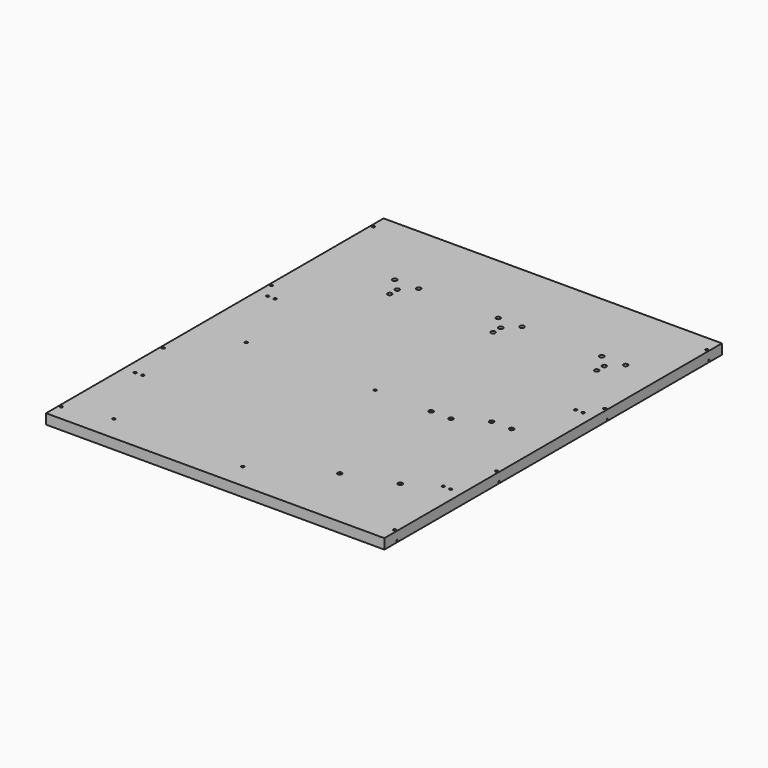
from build123d import *

# Parameters (mm, degrees)
F0_W            = 425
F0_H            = 530
F1_DEPTH        = 6.35
F3_D            = 3.3
F3_CBORE_D      = 6.5
F3_CBORE_DEPTH  = 3
F5_D            = 5.5
F5_CBORE_D      = 9.75
F5_CBORE_DEPTH  = 5
F7_D            = 3.3
F7_CBORE_D      = 6.5
F7_CBORE_DEPTH  = 3
F9_D            = 5.5
F9_DEPTH        = 1
F9_TIP          = 1.6523667023
F11_D           = 3.3
F11_CBORE_D     = 6.5
F11_CBORE_DEPTH = 3


# Not quite as in the source:
# - a feature names something its author has since deleted; it is built from what else it names


with BuildPart() as f1:
    # F0 (on Top) → F1 (new body, symmetric)
    with BuildSketch(Plane.XY):
        Rectangle(F0_W, F0_H)
    extrude(amount=F1_DEPTH, both=True)

    # F3 (through all)
    with Locations(Plane(origin=(0, 0, -6.35), x_dir=(1, 0, 0), z_dir=(0, 0, -1))):
        with Locations((-209.325, 245), (-209.325, 85), (-209.325, -85), (-209.325, -245), (209.325, -245), (209.325, -85), (209.325, 85), (209.325, 245), (-198.2, 143), (-188.7, 143), (198.2, 143), (188.7, 143), (-198.2, -65), (-188.7, -65), (188.7, -65), (198.2, -65)):
            CounterBoreHole(F3_D / 2, F3_CBORE_D / 2, F3_CBORE_DEPTH)

    # F5 (through all)
    with Locations(Plane(origin=(0, 0, -6.35), x_dir=(1, 0, 0), z_dir=(0, 0, -1))):
        with Locations((-122.5, -170), (-92.5, -170), (-107.5, -155.235), (-107.5, -143.235), (167.5, -170), (152.5, -155.235), (152.5, -143.235), (137.5, -170), (37.5, -170), (7.5, -170), (22.5, -155.235), (22.5, -143.235)):
            CounterBoreHole(F5_D / 2, F5_CBORE_D / 2, F5_CBORE_DEPTH)

    # F7 (through all)
    with Locations(Plane(origin=(0, 0, -6.35), x_dir=(1, 0, 0), z_dir=(0, 0, -1))):
        with Locations((152.5, 165), (165, 6), (140, 6), (92.5, 185), (105, 26), (80, 26)):
            CounterBoreHole(F7_D / 2, F7_CBORE_D / 2, F7_CBORE_DEPTH)

    # F9
    with Locations(Plane.XY.offset(6.35)):
        with Locations((165, -6), (140, -6), (105, -26), (105, -26), (80, -26), (152.5, -165), (92.5, -185)):
            Hole(F9_D / 2, depth=F9_DEPTH)
            with Locations((0, 0, -(F9_DEPTH + F9_TIP / 2))):  # 118° drill point
                Cone(0, F9_D / 2, F9_TIP, mode=Mode.SUBTRACT)

    # F11 (through all)
    with Locations(Plane(origin=(0, 0, -6.35), x_dir=(1, 0, 0), z_dir=(0, 0, -1))):
        with Locations((-153, 233), (9, 233), (9, 25), (-153, 25)):
            CounterBoreHole(F11_D / 2, F11_CBORE_D / 2, F11_CBORE_DEPTH)


solid = f1.part
